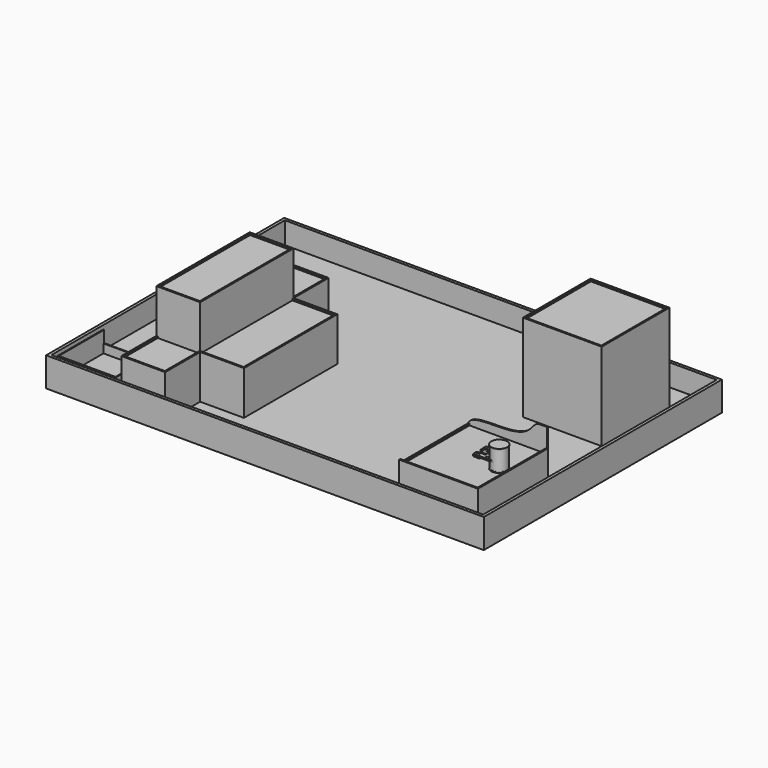
from build123d import *

# Parameters (mm, degrees)
F0_R      = 27.2
F1_DEPTH  = 2.83
F2_R      = 26.4
F3_DEPTH  = 67.36
F4_R      = 27.2
F5_DEPTH  = 2.83
F9_W      = 270
F9_H      = 300
F10_DEPTH = 72
F12_DEPTH = 15
F14_DEPTH = 5
F15_W     = 5
F15_H     = 290
F16_DEPTH = 5
F17_W     = 1500
F17_H     = 1020
F18_DEPTH = 25
F19_W     = 270
F19_H     = 290
F20_DEPTH = 300
F21_W     = 260
F21_H     = 280
F22_DEPTH = 5
F23_W     = 1500
F23_H     = 1020
F23_W_2   = 1480
F23_H_2   = 1000
F24_DEPTH = 75
F26_DEPTH = 150
F27_W     = 150
F27_H     = 400
F28_DEPTH = 150
F29_W     = 140
F29_H     = 390
F30_DEPTH = 5
F31_W     = 140
F31_H     = 145
F31_W_2   = 145
F31_H_2   = 390
F32_DEPTH = 5
F33_R     = 3
F34_DEPTH = 4
F35_R     = 3.99999
F35_2_R   = 3.99999
F36_R     = 3
F37_DEPTH = 8
F38_R     = 3
F39_DEPTH = 8
F40_R     = 3
F40_R_2   = 2.5
F41_DEPTH = 3
F42_R     = 3
F42_R_2   = 2.5
F43_DEPTH = 3
F45_DEPTH = 270.001
F46_W     = 200
F46_H     = 200
F46_W_2   = 194
F46_H_2   = 191
F47_DEPTH = 30
F49_DEPTH = 40
F50_R     = 2.5
F51_DEPTH = 5
F52_R     = 5


# Not quite as in the source:
# - a fillet or chamfer is up to 0.001 mm smaller than in the source, because OpenCascade refuses the exact size
# - a feature names something its author has since deleted; it is built from what else it names


with BuildPart() as f1:
    # F0 (on Top) → F1 (new body)
    with BuildSketch(Plane.XY):
        Circle(F0_R)
    extrude(amount=F1_DEPTH)

    # F2 (on face) → F3 (join)
    with BuildSketch(Plane.XY.offset(2.83)):
        Circle(F2_R)
    extrude(amount=F3_DEPTH)

    # F4 (on face) → F5 (join)
    with BuildSketch(Plane.XY.offset(70.19)):
        Circle(F4_R)
    extrude(amount=F5_DEPTH)


with BuildPart() as f10:
    # F9 (on Top) → F10 (new body)
    with BuildSketch(Plane.XY):
        with Locations((-87.8, 0)):
            Rectangle(F9_W, F9_H)
    extrude(amount=-F10_DEPTH)

    # F11 (on face) → F12 (join)
    with BuildSketch(Plane.XY):
        Polygon((-222.8, -145), (-222.8, -150), (47.2, -150), (47.2, 150), (42.2, 150), (42.2, -145), align=None)
    extrude(amount=F12_DEPTH)

    # F13 (on face) → F14 (join)
    with BuildSketch(Plane(origin=(0, 150, 0), x_dir=(-1, 0, 0), z_dir=(0, 1, 0))):
        with BuildLine():
            Line((-21.3134280931, 81.3575685024), (-47.2, 81.3575685024))
            Line((-47.2, 81.3575685024), (-47.2, -72))
            Line((-47.2, -72), (222.8, -72))
            Line((222.8, -72), (222.8, 0))
            add(Edge.make_bspline(
                [(-21.3134280931, 81.3575685024), (-6.3059147253, 81.3822787863), (12.9585432644, 38.1268753575), (103.6097013063, 23.6068887567), (223.0224295336, 30.7718731823), (222.8, 0)],
                knots=[0, 0, 0, 0, 0.2487100673, 0.6151112321, 1, 1, 1, 1], degree=3))
        make_face()
    extrude(amount=-F14_DEPTH)

    # F15 (on face) → F16 (join)
    with BuildSketch(Plane.XY):
        with Locations((-220.3, 0)):
            Rectangle(F15_W, F15_H)
    extrude(amount=F16_DEPTH)

    # F17 (on face) → F18 (join)
    with BuildSketch(Plane(origin=(0, 0, -72), x_dir=(1, 0, 0), z_dir=(0, 0, -1))):
        with Locations((-602.8, -260)):
            Rectangle(F17_W, F17_H)
    extrude(amount=F18_DEPTH)

    # F19 (on face) → F20 (join)
    with BuildSketch(Plane.XY.offset(-72)):
        with Locations((-87.8, 525)):
            Rectangle(F19_W, F19_H)
    extrude(amount=F20_DEPTH)

    # F21 (on face) → F22 (cut)
    with BuildSketch(Plane.XY.offset(228)):
        with Locations((-87.8, 525)):
            Rectangle(F21_W, F21_H)
    extrude(amount=-F22_DEPTH, mode=Mode.SUBTRACT)

    # F23 (on face) → F24 (join)
    with BuildSketch(Plane.XY.offset(-72)):
        with Locations((-602.8, 260)):
            Rectangle(F23_W, F23_H)
        with Locations((-602.8, 260)):
            Rectangle(F23_W_2, F23_H_2, mode=Mode.SUBTRACT)
    extrude(amount=F24_DEPTH)

    # F25 (on face) → F26 (join)
    with BuildSketch(Plane.XY.offset(-72)):
        Polygon((-952.8, 460), (-1102.8, 460), (-1102.8, -240), (-952.8, -240), (-952.8, -90), (-802.8, -90), (-802.8, 310), (-952.8, 310), align=None)
    extrude(amount=F26_DEPTH)

    # F27 (on face) → F28 (join)
    with BuildSketch(Plane.XY.offset(78)):
        with Locations((-1027.8, 110)):
            Rectangle(F27_W, F27_H)
    extrude(amount=F28_DEPTH)

    # F29 (on face) → F30 (cut)
    with BuildSketch(Plane.XY.offset(228)):
        with Locations((-1027.8, 110)):
            Rectangle(F29_W, F29_H)
    extrude(amount=-F30_DEPTH, mode=Mode.SUBTRACT)

    # F31 (on face) → F32 (cut)
    with BuildSketch(Plane.XY.offset(78)):
        with Locations((-1027.8, 382.5)):
            Rectangle(F31_W, F31_H)
        with Locations((-880.3, 110)):
            Rectangle(F31_W_2, F31_H_2)
        with Locations((-1027.8, -162.5)):
            Rectangle(F31_W, F31_H)
    extrude(amount=-F32_DEPTH, mode=Mode.SUBTRACT)

    # F46 (on face) → F47 (join)
    with BuildSketch(Plane.XY.offset(-72)):
        with Locations((-1232.8, -130)):
            Rectangle(F46_W, F46_H)
        with Locations((-1232.8, -128.5)):
            Rectangle(F46_W_2, F46_H_2, mode=Mode.SUBTRACT)
    extrude(amount=F47_DEPTH)

    # F48 (on face) → F49 (join)
    with BuildSketch(Plane.XY.offset(-42)):
        Polygon((-1329.8, -30), (-1332.8, -30), (-1332.8, -230), (-1329.8, -230), (-1135.8, -230), (-1132.8, -230), (-1132.8, -30), (-1135.8, -30), (-1135.8, -224), (-1329.8, -224), align=None)
    extrude(amount=F49_DEPTH)


with BuildPart() as f34:
    # F33 (on offset) → F34 (new body, symmetric)
    with BuildSketch(Plane.XY.offset(25)):
        with BuildLine():
            Line((-55, -12), (-74.5, -12))
            Line((-74.5, -12), (-74.5, -13))
            Line((-74.5, -13), (-65.6457513111, -13))
            ThreePointArc((-65.6457513111, -13), (-67, -16), (-65.6457513111, -19))
            Line((-65.6457513111, -19), (-74.5, -19))
            Line((-74.5, -19), (-74.5, -20))
            Line((-74.5, -20), (-55, -20))
            ThreePointArc((-55, -20), (-51, -16), (-55, -12))
        make_face()
        with Locations((-63, -16)):
            Circle(F33_R, mode=Mode.SUBTRACT)
        with Locations((-55, -16)):
            Circle(F33_R, mode=Mode.SUBTRACT)
    extrude(amount=F34_DEPTH, both=True)

    # F35 (radius 4 in the source; OpenCascade refuses exactly that, so slightly less here)
    f35_edges = [f34.edges().sort_by_distance(p)[0] for p in [
        (-74.5, -19.5, 29),
        (-74.5, -12.5, 29),
        (-74.5, -19.5, 21),
        (-74.5, -12.5, 21),
    ]]
    fillet(f35_edges, radius=F35_R)

    # F36 (on face) → F37 (join, through all)
    with BuildSketch(Plane.XZ.offset(20)):
        with Locations((-70.5, 25)):
            Circle(F36_R)
    extrude(amount=-F37_DEPTH)

    # F42 (on offset) → F43 (join, symmetric)
    with BuildSketch(Plane.XY.offset(25)):
        with Locations((-63, -16)):
            Circle(F42_R)
        with Locations((-63, -16)):
            Circle(F42_R_2, mode=Mode.SUBTRACT)
        with Locations((-55, -16)):
            Circle(F42_R)
        with Locations((-55, -16)):
            Circle(F42_R_2, mode=Mode.SUBTRACT)
    extrude(amount=F43_DEPTH, both=True)


with BuildPart() as f34b:
    # F33 (on offset) → F34, piece 2 (new body, symmetric)
    with BuildSketch(Plane.XY.offset(25)):
        with BuildLine():
            Line((-74.5, 13), (-74.5, 12))
            Line((-74.5, 12), (-55, 12))
            ThreePointArc((-55, 12), (-51, 16), (-55, 20))
            Line((-55, 20), (-74.5, 20))
            Line((-74.5, 20), (-74.5, 19))
            Line((-74.5, 19), (-65.6457513111, 19))
            ThreePointArc((-65.6457513111, 19), (-67, 16), (-65.6457513111, 13))
            Line((-65.6457513111, 13), (-74.5, 13))
        make_face()
        with Locations((-63, 16)):
            Circle(F33_R, mode=Mode.SUBTRACT)
        with Locations((-55, 16)):
            Circle(F33_R, mode=Mode.SUBTRACT)
    extrude(amount=F34_DEPTH, both=True)

    # F35#2 (radius 4 in the source; OpenCascade refuses exactly that, so slightly less here)
    f35_2_edges = [f34b.edges().sort_by_distance(p)[0] for p in [
        (-74.5, 12.5, 29),
        (-74.5, 19.5, 29),
        (-74.5, 19.5, 21),
        (-74.5, 12.5, 21),
    ]]
    fillet(f35_2_edges, radius=F35_2_R)

    # F38 (on face) → F39 (join, through all)
    with BuildSketch(Plane(origin=(0, 20, 0), x_dir=(-1, 0, 0), z_dir=(0, 1, 0))):
        with Locations((70.5, 25)):
            Circle(F38_R)
    extrude(amount=-F39_DEPTH)

    # F40 (on offset) → F41 (join, symmetric)
    with BuildSketch(Plane.XY.offset(25)):
        with Locations((-55, 16)):
            Circle(F40_R)
        with Locations((-55, 16)):
            Circle(F40_R_2, mode=Mode.SUBTRACT)
        with Locations((-63, 16)):
            Circle(F40_R)
        with Locations((-63, 16)):
            Circle(F40_R_2, mode=Mode.SUBTRACT)
    extrude(amount=F41_DEPTH, both=True)


with BuildPart() as f45_tool:
    # F44 (on face) → F45 (new body, through all)
    with BuildSketch(Plane(origin=(0, 20, 0), x_dir=(-1, 0, 0), z_dir=(0, 1, 0))):
        with BuildLine():
            Line((71.5, 26), (71.5, 27.2912878475))
            ThreePointArc((71.5, 27.2912878475), (70.5, 27.5), (69.5, 27.2912878475))
            Line((69.5, 27.2912878475), (69.5, 26))
            Line((69.5, 26), (68.2087121525, 26))
            ThreePointArc((68.2087121525, 26), (68, 25), (68.2087121525, 24))
            Line((68.2087121525, 24), (69.5, 24))
            Line((69.5, 24), (69.5, 22.7087121525))
            ThreePointArc((69.5, 22.7087121525), (70.5, 22.5), (71.5, 22.7087121525))
            Line((71.5, 22.7087121525), (71.5, 24))
            Line((71.5, 24), (72.7912878475, 24))
            ThreePointArc((72.7912878475, 24), (73, 25), (72.7912878475, 26))
            Line((72.7912878475, 26), (71.5, 26))
        make_face()
    extrude(amount=-F45_DEPTH)


with BuildPart() as f34_1:
    add(f34.part)

    # F45: cut by f45_tool
    add(f45_tool.part, mode=Mode.SUBTRACT)


with BuildPart() as f34b_1:
    add(f34b.part)

    # F45: cut by f45_tool
    add(f45_tool.part, mode=Mode.SUBTRACT)


with BuildPart() as f51:
    # F50 (on face) → F51 (new body)
    with BuildSketch(Plane.XY.offset(29)):
        with BuildLine():
            Line((0.3855752584, 27.1972669899), (0.3855752584, 27.2667966783))
            Line((0.3855752584, 27.2667966783), (-67.0419484377, 27.2667966783))
            Line((-67.0419484377, 27.2667966783), (-67.0419484377, 12))
            Line((-67.0419484377, 12), (-37.6948826015, 12))
            Line((-37.6948826015, 12), (-37.6948826015, -12))
            Line((-37.6948826015, -12), (-67.0419484377, -12))
            Line((-67.0419484377, -12), (-67.0419484377, -27.4200625718))
            Line((-67.0419484377, -27.4200625718), (0.3855752584, -27.4200625718))
            Line((0.3855752584, -27.4200625718), (0.3855752584, -27.1972669899))
            ThreePointArc((0.3855752584, -27.1972669899), (-27.2, 0), (0.3855752584, 27.1972669899))
        make_face()
        with Locations((-63, -16)):
            Circle(F50_R, mode=Mode.SUBTRACT)
        with Locations((-55, -16)):
            Circle(F50_R, mode=Mode.SUBTRACT)
        with Locations((-27.3543447256, -19.4251015782)):
            Circle(F50_R, mode=Mode.SUBTRACT)
        with Locations((-63, 16)):
            Circle(F50_R, mode=Mode.SUBTRACT)
        with Locations((-55, 16)):
            Circle(F50_R, mode=Mode.SUBTRACT)
        with Locations((-32.8015722334, 0)):
            Circle(F50_R, mode=Mode.SUBTRACT)
        with Locations((-27.3543447256, 19.4251015782)):
            Circle(F50_R, mode=Mode.SUBTRACT)
        with BuildLine():
            Line((0.3855752584, 27.1972669899), (0.3855752584, 27.2667966783))
            Line((0.3855752584, 27.2667966783), (-67.0419484377, 27.2667966783))
            Line((-67.0419484377, 27.2667966783), (-67.0419484377, 12))
            Line((-67.0419484377, 12), (-37.6948826015, 12))
            Line((-37.6948826015, 12), (-37.6948826015, -12))
            Line((-37.6948826015, -12), (-55, -12))
            ThreePointArc((-55, -12), (-51, -16), (-55, -20))
            Line((-55, -20), (-67.0419484377, -20))
            Line((-67.0419484377, -20), (-67.0419484377, -27.4200625718))
            Line((-67.0419484377, -27.4200625718), (0.3855752584, -27.4200625718))
            Line((0.3855752584, -27.4200625718), (0.3855752584, -27.1972669899))
            ThreePointArc((0.3855752584, -27.1972669899), (-27.2, 0), (0.3855752584, 27.1972669899))
        make_face()
        with Locations((-27.3543447256, -19.4251015782)):
            Circle(F50_R, mode=Mode.SUBTRACT)
        with Locations((-63, 16)):
            Circle(F50_R, mode=Mode.SUBTRACT)
        with Locations((-55, 16)):
            Circle(F50_R, mode=Mode.SUBTRACT)
        with Locations((-32.8015722334, 0)):
            Circle(F50_R, mode=Mode.SUBTRACT)
        with Locations((-27.3543447256, 19.4251015782)):
            Circle(F50_R, mode=Mode.SUBTRACT)
    extrude(amount=F51_DEPTH)

    # F52
    f52_edges = [f51.edges().sort_by_distance(p)[0] for p in [
        (-37.694883, 12, 31.5),
        (-37.694883, -12, 31.5),
        (-67.041948, 27.266797, 31.5),
        (-67.041948, 12, 31.5),
        (-67.041948, -27.420063, 31.5),
        (-67.041948, -12, 31.5),
    ]]
    fillet(f52_edges, radius=F52_R)


solid = Compound([f1.part, f10.part, f34_1.part, f34b_1.part, f51.part])
